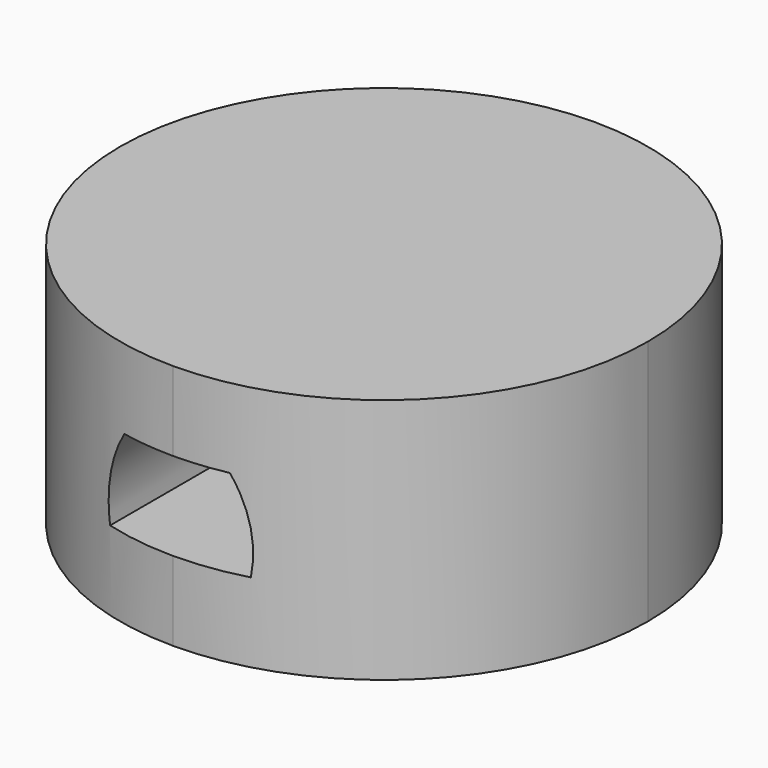
from build123d import *

# Parameters (mm, degrees)
F0_W        = 15
F0_H        = 15
F1_DEPTH    = 7
F3_DEPTH    = 10.6
F4_T1_DEPTH = 44.5


# Not quite as in the source:
# - a fillet or chamfer that OpenCascade refuses, or shapes differently, is made with other operations: its cross-section is extruded or revolved along the edge and cut away or added


with BuildPart() as f1:
    # F0 (on Top) → F1 (new body)
    with BuildSketch(Plane.XY):
        Rectangle(F0_W, F0_H)
    extrude(amount=F1_DEPTH)

    # F2 (on face) → F3 (cut)
    with BuildSketch(Plane.XZ.offset(7.5)):
        with BuildLine():
            ThreePointArc((2, 2.25), (1.9853102837, 3.5470620567), (1.5, 4.75))
            Line((1.5, 4.75), (-1.5, 4.75))
            ThreePointArc((-1.5, 4.75), (-1.9853102837, 3.5470620567), (-2, 2.25))
            Line((-2, 2.25), (2, 2.25))
        make_face()
    extrude(amount=-F3_DEPTH, mode=Mode.SUBTRACT)

    # F4: fillet of radius 7.5 on 4 edges, made by hand

    # F4_s2 → F4_t1 (cut)
    with BuildSketch(Plane.XY.offset(-18.75)):
        with BuildLine():
            ThreePointArc((0, -7.5), (-5.3033008589, -5.3033008589), (-7.5, 0))
            Line((-7.5, 0), (-7.5, -7.5))
            Line((-7.5, -7.5), (0, -7.5))
        make_face()
        with BuildLine():
            ThreePointArc((0, -7.5), (5.3033008589, -5.3033008589), (7.5, 0))
            Line((7.5, 0), (7.5, -7.5))
            Line((7.5, -7.5), (0, -7.5))
        make_face()
        with BuildLine():
            ThreePointArc((7.5, 0), (5.3033008589, 5.3033008589), (0, 7.5))
            Line((0, 7.5), (7.5, 7.5))
            Line((7.5, 7.5), (7.5, 0))
        make_face()
        with BuildLine():
            ThreePointArc((-7.5, 0), (-5.3033008589, 5.3033008589), (0, 7.5))
            Line((0, 7.5), (-7.5, 7.5))
            Line((-7.5, 7.5), (-7.5, 0))
        make_face()
    extrude(amount=F4_T1_DEPTH, mode=Mode.SUBTRACT)


solid = f1.part
